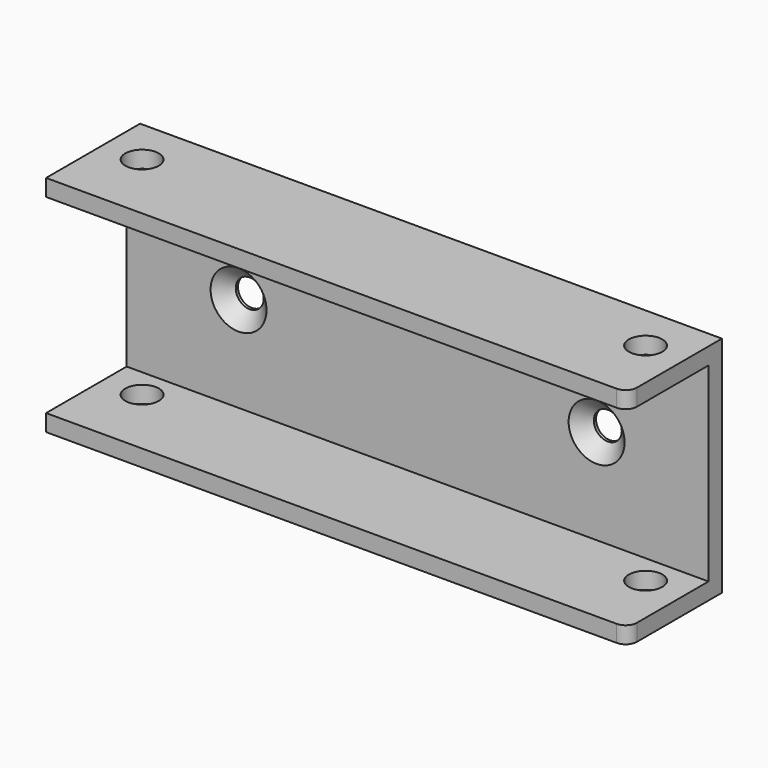
from build123d import *

# Parameters (mm, degrees)
F0_W     = 104
F0_H     = 3
F1_DEPTH = 21
F0_H_2   = 34
F0_R     = 2.5
F2_DEPTH = 3
F4_D     = 6
F5_SIZE  = 2.5
F6_SIZE  = 2.5
F7_R     = 2


with BuildPart() as f1:
    # F0 (on Front) → F1 (new body)
    with BuildSketch(Plane.XZ):
        with Locations((0, 18.5)):
            Rectangle(F0_W, F0_H)
    extrude(amount=F1_DEPTH)



with BuildPart() as f1b:
    # F0 (on Front) → F1, piece 2 (new body)
    with BuildSketch(Plane.XZ):
        with Locations((0, -18.5)):
            Rectangle(F0_W, F0_H)
    extrude(amount=F1_DEPTH)


with BuildPart() as f1_1:
    add(f1.part)

    add(f1b.part)  # F2 merges F1b
    # F0 (on Front) → F2 (join)
    with BuildSketch(Plane.XZ):
        Rectangle(F0_W, F0_H_2)
        with Locations((-32, 0)):
            Circle(F0_R, mode=Mode.SUBTRACT)
        with Locations((32, 0)):
            Circle(F0_R, mode=Mode.SUBTRACT)
    extrude(amount=F2_DEPTH)

    # F4 (through all)
    with Locations(Plane(origin=(0, 0, -20), x_dir=(1, 0, 0), z_dir=(0, 0, -1))):
        with Locations((-45, 8.3), (45, 8.2999998429)):
            Hole(F4_D / 2)

    # F5
    f5_edges = [f1_1.edges().sort_by_distance(p)[0] for p in [
        (-34.5, -3, 0),
    ]]
    chamfer(f5_edges, length=F5_SIZE)

    # F6
    f6_edges = [f1_1.edges().sort_by_distance(p)[0] for p in [
        (29.5, -3, 0),
    ]]
    chamfer(f6_edges, length=F6_SIZE)

    # F7
    f7_edges = [f1_1.edges().sort_by_distance(p)[0] for p in [
        (52, -21, -18.5),
        (52, -21, 18.5),
    ]]
    fillet(f7_edges, radius=F7_R)


solid = f1_1.part
